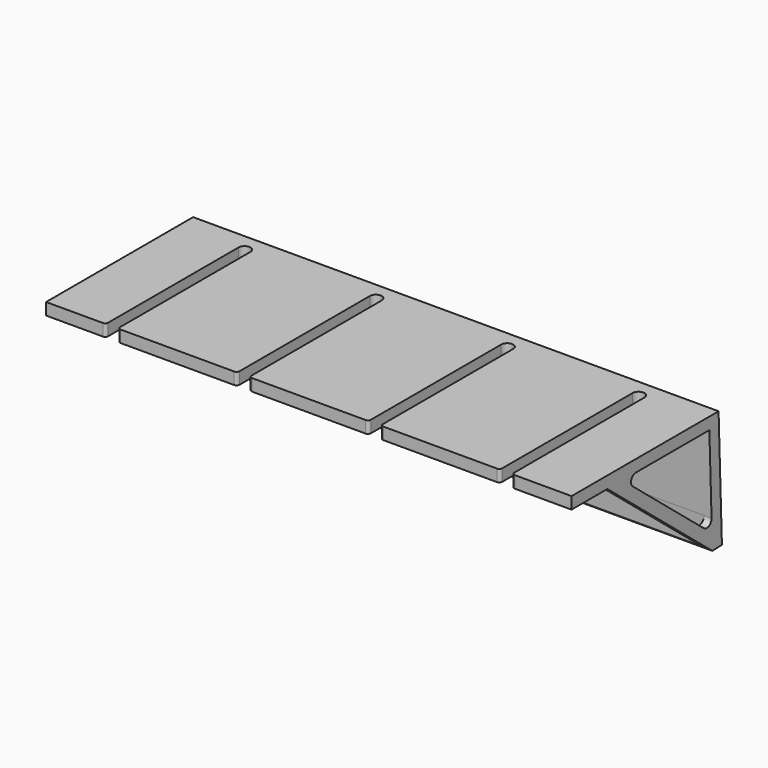
from build123d import *

# Parameters (mm, degrees)
F1_DEPTH = 4
F4_DEPTH = 176
F6_W     = 40.25
F6_H     = 35.9756330808
F6_W_2   = 41.5
F7_REACH = 113.8761797882
F8_R     = 2
F9_DEPTH = 25


# Not quite as in the source:
# - a feature names something its author has since deleted; it is built from what else it names


with BuildPart() as f1:
    # F0 (on Top) → F1 (new body)
    with BuildSketch(Plane.XY):
        with BuildLine():
            Line((176, 0), (0, 0))
            Line((0, 0), (0, -61.56))
            Line((0, -61.56), (19, -61.56))
            ThreePointArc((19, -61.56), (19.7071067812, -61.2671067812), (20, -60.56))
            Line((20, -60.56), (20, -6))
            ThreePointArc((20, -6), (22, -4), (24, -6))
            Line((24, -6), (24, -60.56))
            ThreePointArc((24, -60.56), (24.2928932188, -61.2671067812), (25, -61.56))
            Line((25, -61.56), (63, -61.56))
            ThreePointArc((63, -61.56), (63.7071067812, -61.2671067812), (64, -60.56))
            Line((64, -60.56), (64, -6))
            ThreePointArc((64, -6), (66, -4), (68, -6))
            Line((68, -6), (68, -60.56))
            ThreePointArc((68, -60.56), (68.2928932188, -61.2671067812), (69, -61.56))
            Line((69, -61.56), (107, -61.56))
            ThreePointArc((107, -61.56), (107.7071067812, -61.2671067812), (108, -60.56))
            Line((108, -60.56), (108, -6))
            ThreePointArc((108, -6), (110, -4), (112, -6))
            Line((112, -6), (112, -60.56))
            ThreePointArc((112, -60.56), (112.2928932188, -61.2671067812), (113, -61.56))
            Line((113, -61.56), (151, -61.56))
            ThreePointArc((151, -61.56), (151.7071067812, -61.2671067812), (152, -60.56))
            Line((152, -60.56), (152, -6))
            ThreePointArc((152, -6), (154, -4), (156, -6))
            Line((156, -6), (156, -60.56))
            ThreePointArc((156, -60.56), (156.2928932188, -61.2671067812), (157, -61.56))
            Line((157, -61.56), (176, -61.56))
            Line((176, -61.56), (176, 0))
        make_face()
    extrude(amount=F1_DEPTH)

    # F3 (on face) → F4 (join, through all)
    with BuildSketch(Plane(origin=(0, 0, 0), x_dir=(0, -1, 0), z_dir=(-1, 0, 0))):
        with BuildLine():
            Line((2.9423112754, -26.3580624732), (3.8627550992, 0))
            Line((3.8627550992, 0), (0, 0))
            Line((0, 0), (0, 4))
            Line((0, 4), (-1.3959798681, -35.9756330808))
            Line((-1.3959798681, -35.9756330808), (2.60158344, -36.1152310676))
            Line((2.60158344, -36.1152310676), (46.56, 0))
            Line((46.56, 0), (34.6739806412, 0))
            ThreePointArc((34.6739806412, 0), (36.5568879354, -1.3257151036), (35.9435965909, -3.5453398785))
            Line((35.9435965909, -3.5453398785), (6.2107088791, -27.9732013451))
            ThreePointArc((6.2107088791, -27.9732013451), (4.0550404197, -28.220878742), (2.9423112754, -26.3580624732))
        make_face()
    extrude(amount=-F4_DEPTH)

    f7_end = Plane(origin=(88, -3.299573374, -16.1274145272), x_dir=(0, -0.0348994967, 0.999390827), z_dir=(0, 0.999390827, 0.0348994967))
    # F6 (on face) → F7 (cut, up to a plane its end follows)
    with BuildSketch(Plane.XZ.offset(61.56)):
        with Locations((153.375, -17.9878165404)):
            Rectangle(F6_W, F6_H)
        with Locations((110, -17.9878165404)):
            Rectangle(F6_W_2, F6_H)
        with Locations((66, -17.9878165404)):
            Rectangle(F6_W_2, F6_H)
        Polygon((19, 0), (2.5, 0), (2.5, -35.9756330808), (42.75, -35.9756330808), (42.75, 0), align=None)
    f7_long = extrude(amount=-F7_REACH, mode=Mode.PRIVATE)
    add(split(f7_long, bisect_by=f7_end, keep=Keep.BOTTOM, mode=Mode.PRIVATE), mode=Mode.SUBTRACT)

    # F8 (on face) → F9 (cut)
    with BuildSketch(Plane(origin=(0, 0.1395129475, 0.0048718995), x_dir=(-1, 0, 0), z_dir=(0, 0.999390827, 0.0348994967))):
        with Locations((-147.0000000001, -16.0024366919)):
            Circle(F8_R)
        with Locations((-21, -16.0024366919)):
            Circle(F8_R)
    extrude(amount=-F9_DEPTH, mode=Mode.SUBTRACT)


solid = f1.part
